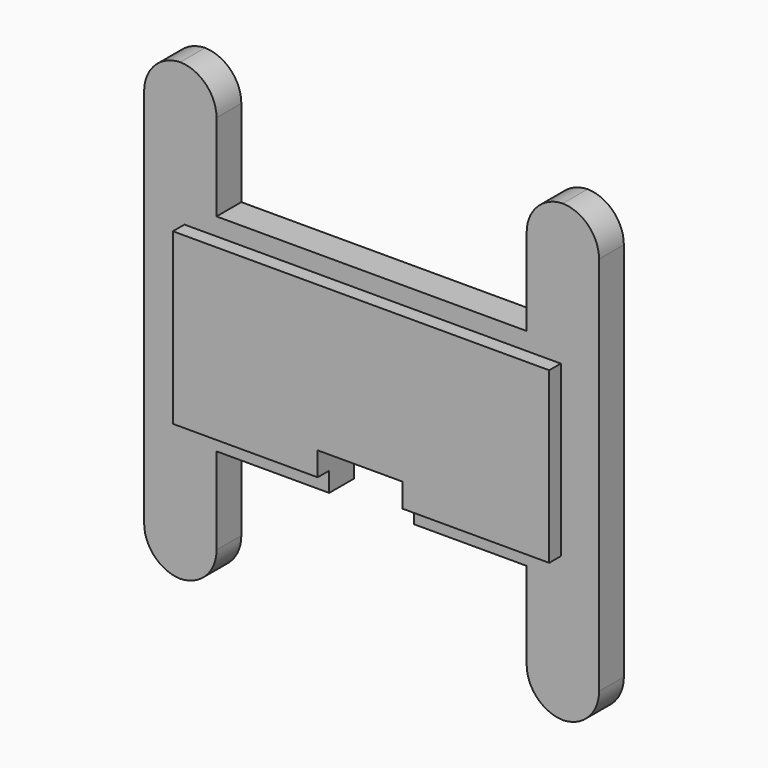
from build123d import *

# Parameters (mm, degrees)
F0_W         = 55.88
F0_H         = 25.4
F1_DEPTH     = 3.81
F2_W         = 46.228
F2_H         = 20.828
F3_DEPTH     = 1.778
F4_W         = 10.414
F4_H         = 9.1227373774
F5_DEPTH     = 25.4
F6_W         = 8.89
F6_H         = 15.24
F7_DEPTH     = 3.81
F8_T1_DEPTH  = 26.67
F10_W        = 8.89
F10_H        = 15.24
F11_DEPTH    = 3.81
F12_T1_DEPTH = 26.67
F13_W        = 8.89
F13_H        = 15.24
F14_DEPTH    = 3.81
F15_T1_DEPTH = 26.67
F16_W        = 8.89
F16_H        = 15.24
F17_DEPTH    = 3.81
F18_T1_DEPTH = 26.67


# Not quite as in the source:
# - a fillet or chamfer that OpenCascade refuses, or shapes differently, is made with other operations: its cross-section is extruded or revolved along the edge and cut away or added


with BuildPart() as f1:
    # F0 (on Front) → F1 (new body)
    with BuildSketch(Plane.XZ):
        with Locations((8.0322436088, 0.5406907029)):
            Rectangle(F0_W, F0_H)
    extrude(amount=F1_DEPTH)

    # F2 (on face) → F3 (join)
    with BuildSketch(Plane.XZ.offset(3.81)):
        with Locations((8.1592436088, 0.6676907029)):
            Rectangle(F2_W, F2_H)
    extrude(amount=F3_DEPTH)

    # F4 (on face) → F5 (cut)
    with BuildSketch(Plane.XZ):
        with Locations((8.0322436088, -11.3866779858)):
            Rectangle(F4_W, F4_H)
    extrude(amount=F5_DEPTH, mode=Mode.SUBTRACT)

    # F6 (on face) → F7 (join)
    with BuildSketch(Plane.XZ):
        with Locations((31.5272436088, 20.8606907029)):
            Rectangle(F6_W, F6_H)
    extrude(amount=F7_DEPTH)

    # F8: fillet of radius 4.572 on 2 edges, made by hand

    # F8_s2 → F8_t1 (cut)
    with BuildSketch(Plane.XZ.offset(-11.43)):
        with BuildLine():
            ThreePointArc((31.4002436088, 28.4806907029), (34.6331358124, 27.1415829065), (35.9722436088, 23.9086907029))
            Line((35.9722436088, 23.9086907029), (35.9722436088, 28.4806907029))
            Line((35.9722436088, 28.4806907029), (31.4002436088, 28.4806907029))
        make_face()
        with BuildLine():
            ThreePointArc((27.0822436088, 23.9086907029), (28.4213514052, 27.1415829065), (31.6542436088, 28.4806907029))
            Line((31.6542436088, 28.4806907029), (27.0822436088, 28.4806907029))
            Line((27.0822436088, 28.4806907029), (27.0822436088, 23.9086907029))
        make_face()
    extrude(amount=F8_T1_DEPTH, mode=Mode.SUBTRACT)

    # F10 (on face) → F11 (join)
    with BuildSketch(Plane.XZ):
        with Locations((-15.4627563912, 20.8606907029)):
            Rectangle(F10_W, F10_H)
    extrude(amount=F11_DEPTH)

    # F12: fillet of radius 4.572 on 2 edges, made by hand

    # F12_s2 → F12_t1 (cut)
    with BuildSketch(Plane.XZ.offset(-11.43)):
        with BuildLine():
            ThreePointArc((-19.9077563912, 23.9086907029), (-18.5686485948, 27.1415829065), (-15.3357563912, 28.4806907029))
            Line((-15.3357563912, 28.4806907029), (-19.9077563912, 28.4806907029))
            Line((-19.9077563912, 28.4806907029), (-19.9077563912, 23.9086907029))
        make_face()
        with BuildLine():
            ThreePointArc((-15.5897563912, 28.4806907029), (-12.3568641876, 27.1415829065), (-11.0177563912, 23.9086907029))
            Line((-11.0177563912, 23.9086907029), (-11.0177563912, 28.4806907029))
            Line((-11.0177563912, 28.4806907029), (-15.5897563912, 28.4806907029))
        make_face()
    extrude(amount=F12_T1_DEPTH, mode=Mode.SUBTRACT)

    # F13 (on face) → F14 (join)
    with BuildSketch(Plane.XZ):
        with Locations((31.5272436088, -19.7793092971)):
            Rectangle(F13_W, F13_H)
    extrude(amount=F14_DEPTH)

    # F15: fillet of radius 4.572 on 2 edges, made by hand

    # F15_s2 → F15_t1 (cut)
    with BuildSketch(Plane.XZ.offset(-11.43)):
        with BuildLine():
            ThreePointArc((35.9722436088, -22.8273092971), (34.6331358124, -26.0602015007), (31.4002436088, -27.3993092971))
            Line((31.4002436088, -27.3993092971), (35.9722436088, -27.3993092971))
            Line((35.9722436088, -27.3993092971), (35.9722436088, -22.8273092971))
        make_face()
        with BuildLine():
            ThreePointArc((31.6542436088, -27.3993092971), (28.4213514052, -26.0602015007), (27.0822436088, -22.8273092971))
            Line((27.0822436088, -22.8273092971), (27.0822436088, -27.3993092971))
            Line((27.0822436088, -27.3993092971), (31.6542436088, -27.3993092971))
        make_face()
    extrude(amount=F15_T1_DEPTH, mode=Mode.SUBTRACT)

    # F16 (on face) → F17 (join)
    with BuildSketch(Plane.XZ):
        with Locations((-15.4627563912, -19.7793092971)):
            Rectangle(F16_W, F16_H)
    extrude(amount=F17_DEPTH)

    # F18: fillet of radius 4.572 on 2 edges, made by hand

    # F18_s2 → F18_t1 (cut)
    with BuildSketch(Plane.XZ.offset(-11.43)):
        with BuildLine():
            ThreePointArc((-15.3357563912, -27.3993092971), (-18.5686485948, -26.0602015007), (-19.9077563912, -22.8273092971))
            Line((-19.9077563912, -22.8273092971), (-19.9077563912, -27.3993092971))
            Line((-19.9077563912, -27.3993092971), (-15.3357563912, -27.3993092971))
        make_face()
        with BuildLine():
            ThreePointArc((-11.0177563912, -22.8273092971), (-12.3568641876, -26.0602015007), (-15.5897563912, -27.3993092971))
            Line((-15.5897563912, -27.3993092971), (-11.0177563912, -27.3993092971))
            Line((-11.0177563912, -27.3993092971), (-11.0177563912, -22.8273092971))
        make_face()
    extrude(amount=F18_T1_DEPTH, mode=Mode.SUBTRACT)


solid = f1.part
